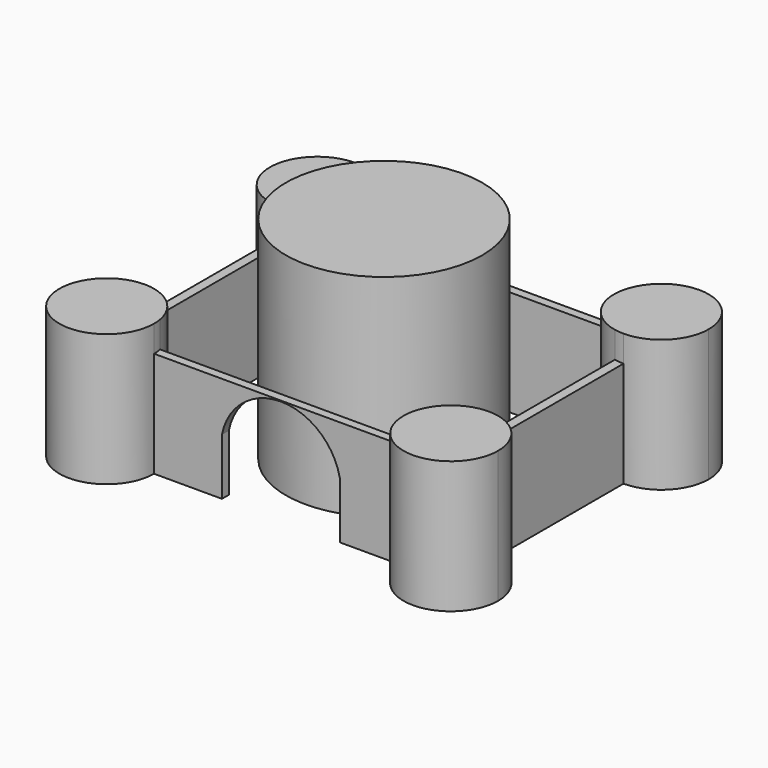
from build123d import *

# Parameters (mm, degrees)
F1_DEPTH = 25.4
F2_DEPTH = 31.75
F0_R     = 23.6132270113
F3_DEPTH = 50.8
F5_DEPTH = 41.91


with BuildPart() as f1:
    # F0 (on Top) → F1 (new body)
    with BuildSketch(Plane.XY):
        with BuildLine():
            Line((29.9722703229, 31.631860882), (-29.9722703229, 31.631860882))
            ThreePointArc((-29.9722703229, 31.631860882), (-30.0197276791, 30.5938091569), (-30.161703811, 29.5644178987))
            Line((-30.161703811, 29.5644178987), (30.161703811, 29.5644178987))
            ThreePointArc((30.161703811, 29.5644178987), (30.0197276791, 30.5938091569), (29.9722703229, 31.631860882))
        make_face()
    extrude(amount=F1_DEPTH)


with BuildPart() as f1b:
    # F0 (on Top) → F1, piece 2 (new body)
    with BuildSketch(Plane.XY):
        with BuildLine():
            Line((-41.348837316, 20.2552938889), (-41.348837316, -20.2552938889))
            ThreePointArc((-41.348837316, -20.2552938889), (-40.2059630767, -20.3128452437), (-39.074651897, -20.4849170305))
            Line((-39.074651897, -20.4849170305), (-39.074651897, 20.4849170305))
            ThreePointArc((-39.074651897, 20.4849170305), (-40.2059630767, 20.3128452437), (-41.348837316, 20.2552938889))
        make_face()
    extrude(amount=F1_DEPTH)


with BuildPart() as f1c:
    # F0 (on Top) → F1, piece 3 (new body)
    with BuildSketch(Plane.XY):
        with BuildLine():
            ThreePointArc((-30.161703811, -29.5644178987), (-30.0197276791, -30.5938091569), (-29.9722703229, -31.631860882))
            Line((-29.9722703229, -31.631860882), (29.9722703229, -31.631860882))
            ThreePointArc((29.9722703229, -31.631860882), (30.0197276791, -30.5938091569), (30.161703811, -29.5644178987))
            Line((30.161703811, -29.5644178987), (-30.161703811, -29.5644178987))
        make_face()
    extrude(amount=F1_DEPTH)

    # F4 (on face) → F5 (cut)
    with BuildSketch(Plane.XZ.offset(31.631860882)):
        with BuildLine():
            Line((-13.6451162398, 13.6451171711), (-13.6451162398, 0))
            Line((-13.6451162398, 0), (14.6788377315, 0))
            Line((14.6788377315, 0), (14.6788377315, 13.6451171711))
            ThreePointArc((14.6788377315, 13.6451171711), (0.5168607458, 25.1843783905), (-13.6451162398, 13.6451171711))
        make_face()
    extrude(amount=-F5_DEPTH, mode=Mode.SUBTRACT)


with BuildPart() as f1d:
    # F0 (on Top) → F1, piece 4 (new body)
    with BuildSketch(Plane.XY):
        with BuildLine():
            Line((39.074651897, 20.4849170305), (39.074651897, -20.4849170305))
            ThreePointArc((39.074651897, -20.4849170305), (40.2059630767, -20.3128452437), (41.348837316, -20.2552938889))
            Line((41.348837316, -20.2552938889), (41.348837316, 20.2552938889))
            ThreePointArc((41.348837316, 20.2552938889), (40.2059630767, 20.3128452437), (39.074651897, 20.4849170305))
        make_face()
    extrude(amount=F1_DEPTH)


with BuildPart() as f2:
    # F0 (on Top) → F2 (new body)
    with BuildSketch(Plane.XY):
        with BuildLine():
            ThreePointArc((-29.9722703229, 31.631860882), (-49.3932849835, 39.6763085495), (-41.348837316, 20.2552938889))
            ThreePointArc((-41.348837316, 20.2552938889), (-40.2059630767, 20.3128452437), (-39.074651897, 20.4849170305))
            ThreePointArc((-39.074651897, 20.4849170305), (-33.2302715069, 23.6622206297), (-30.161703811, 29.5644178987))
            ThreePointArc((-30.161703811, 29.5644178987), (-30.0197276791, 30.5938091569), (-29.9722703229, 31.631860882))
        make_face()
    extrude(amount=F2_DEPTH)


with BuildPart() as f2b:
    # F0 (on Top) → F2, piece 2 (new body)
    with BuildSketch(Plane.XY):
        with BuildLine():
            ThreePointArc((-41.348837316, -20.2552938889), (-49.3932849835, -39.6763085495), (-29.9722703229, -31.631860882))
            ThreePointArc((-29.9722703229, -31.631860882), (-30.0197276791, -30.5938091569), (-30.161703811, -29.5644178987))
            ThreePointArc((-30.161703811, -29.5644178987), (-33.2302715069, -23.6622206297), (-39.074651897, -20.4849170305))
            ThreePointArc((-39.074651897, -20.4849170305), (-40.2059630767, -20.3128452437), (-41.348837316, -20.2552938889))
        make_face()
    extrude(amount=F2_DEPTH)


with BuildPart() as f2c:
    # F0 (on Top) → F2, piece 3 (new body)
    with BuildSketch(Plane.XY):
        with BuildLine():
            ThreePointArc((30.161703811, -29.5644178987), (30.0197276791, -30.5938091569), (29.9722703229, -31.631860882))
            ThreePointArc((29.9722703229, -31.631860882), (41.348837316, -43.0084278752), (52.7254043092, -31.631860882))
            ThreePointArc((52.7254043092, -31.631860882), (49.3932849835, -23.5874132146), (41.348837316, -20.2552938889))
            ThreePointArc((41.348837316, -20.2552938889), (40.2059630767, -20.3128452437), (39.074651897, -20.4849170305))
            ThreePointArc((39.074651897, -20.4849170305), (33.2302715069, -23.6622206297), (30.161703811, -29.5644178987))
        make_face()
    extrude(amount=F2_DEPTH)


with BuildPart() as f2d:
    # F0 (on Top) → F2, piece 4 (new body)
    with BuildSketch(Plane.XY):
        with BuildLine():
            ThreePointArc((30.161703811, 29.5644178987), (33.2302715069, 23.6622206297), (39.074651897, 20.4849170305))
            ThreePointArc((39.074651897, 20.4849170305), (40.2059630767, 20.3128452437), (41.348837316, 20.2552938889))
            ThreePointArc((41.348837316, 20.2552938889), (49.3932849835, 23.5874132146), (52.7254043092, 31.631860882))
            ThreePointArc((52.7254043092, 31.631860882), (41.348837316, 43.0084278752), (29.9722703229, 31.631860882))
            ThreePointArc((29.9722703229, 31.631860882), (30.0197276791, 30.5938091569), (30.161703811, 29.5644178987))
        make_face()
    extrude(amount=F2_DEPTH)


with BuildPart() as f3:
    # F0 (on Top) → F3 (new body)
    with BuildSketch(Plane.XY):
        Circle(F0_R)
    extrude(amount=F3_DEPTH)


solid = Compound([f1.part, f1b.part, f1c.part, f1d.part, f2.part, f2b.part, f2c.part, f2d.part, f3.part])
